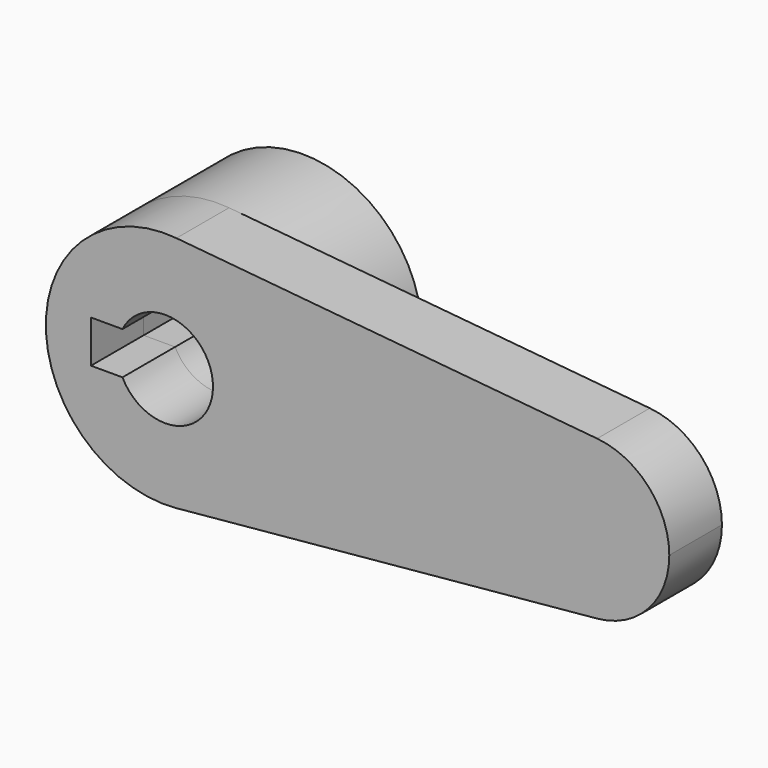
from build123d import *
from build123d import SkipClean  # not in build123d's __all__

# Parameters (mm, degrees)
F0_R     = 11.43
F1_DEPTH = 15.748
F2_DEPTH = 25.4


with BuildPart() as f1:
    # F0 (on Front) → F1 (new body)
    with BuildSketch(Plane.XZ):
        with BuildLine():
            ThreePointArc((2.67890625, 28.4491491315), (21.1314974753, 19.2351355455), (28.575, 0))
            ThreePointArc((28.575, 0), (21.1314974753, -19.2351355455), (2.67890625, -28.4491491315))
            Line((2.67890625, -28.4491491315), (103.3859375, -18.966099421))
            ThreePointArc((103.3859375, -18.966099421), (82.55, 0), (103.3859375, 18.966099421))
            Line((103.3859375, 18.966099421), (2.67890625, 28.4491491315))
        make_face()
        with BuildLine():
            ThreePointArc((2.67890625, -28.4491491315), (21.1314974753, -19.2351355455), (28.575, 0))
            ThreePointArc((28.575, 0), (21.1314974753, 19.2351355455), (2.67890625, 28.4491491315))
            ThreePointArc((2.67890625, 28.4491491315), (-28.575, 0), (2.67890625, -28.4491491315))
        make_face()
        with BuildLine():
            ThreePointArc((-10.2390673403, 5.08), (0, 11.43), (10.2390673403, 5.08))
            Line((10.2390673403, 5.08), (17.78, 5.08))
            Line((17.78, 5.08), (17.78, -5.08))
            Line((17.78, -5.08), (10.2390673403, -5.08))
            ThreePointArc((10.2390673403, -5.08), (0, -11.43), (-10.2390673403, -5.08))
            Line((-10.2390673403, -5.08), (-17.78, -5.08))
            Line((-17.78, -5.08), (-17.78, 5.08))
            Line((-17.78, 5.08), (-10.2390673403, 5.08))
        make_face(mode=Mode.SUBTRACT)
        with BuildLine():
            ThreePointArc((120.65, 0), (115.6876649835, 12.823423697), (103.3859375, 18.966099421))
            ThreePointArc((103.3859375, 18.966099421), (82.55, 0), (103.3859375, -18.966099421))
            ThreePointArc((103.3859375, -18.966099421), (115.6876649835, -12.823423697), (120.65, 0))
        make_face()
        with Locations((101.6, 0)):
            Circle(F0_R, mode=Mode.SUBTRACT)
        with Locations((101.6, 0)):
            Circle(F0_R)
        with BuildLine():
            ThreePointArc((10.2390673403, 5.08), (11.1282846769, 2.6088656826), (11.43, 0))
            ThreePointArc((11.43, 0), (11.1282846769, -2.6088656826), (10.2390673403, -5.08))
            Line((10.2390673403, -5.08), (17.78, -5.08))
            Line((17.78, -5.08), (17.78, 5.08))
            Line((17.78, 5.08), (10.2390673403, 5.08))
        make_face()
    extrude(amount=F1_DEPTH)

    # F0 (on Front) → F2 (join)
    with BuildSketch(Plane.XZ):
        with BuildLine():
            ThreePointArc((2.67890625, -28.4491491315), (21.1314974753, -19.2351355455), (28.575, 0))
            ThreePointArc((28.575, 0), (21.1314974753, 19.2351355455), (2.67890625, 28.4491491315))
            ThreePointArc((2.67890625, 28.4491491315), (-28.575, 0), (2.67890625, -28.4491491315))
        make_face()
        with BuildLine():
            ThreePointArc((-10.2390673403, 5.08), (0, 11.43), (10.2390673403, 5.08))
            Line((10.2390673403, 5.08), (17.78, 5.08))
            Line((17.78, 5.08), (17.78, -5.08))
            Line((17.78, -5.08), (10.2390673403, -5.08))
            ThreePointArc((10.2390673403, -5.08), (0, -11.43), (-10.2390673403, -5.08))
            Line((-10.2390673403, -5.08), (-17.78, -5.08))
            Line((-17.78, -5.08), (-17.78, 5.08))
            Line((-17.78, 5.08), (-10.2390673403, 5.08))
        make_face(mode=Mode.SUBTRACT)
    with SkipClean():  # cleaning this boolean's faces spoils the solid; the shape is the same uncleaned
        extrude(amount=-F2_DEPTH)


solid = f1.part
